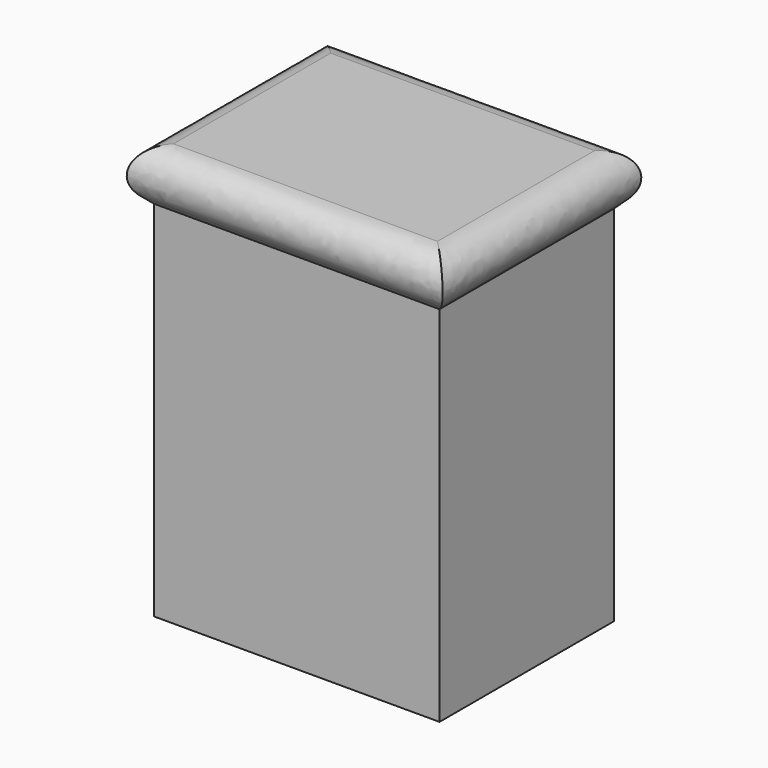
from build123d import *

# Parameters (mm, degrees)
F0_W      = 5.5
F0_H      = 4.2
F1_DEPTH  = 7
F2_W      = 0.8
F2_H      = 0.95
F3_DEPTH  = 5
F1_FACE_W = 5.5
F1_FACE_H = 4.2
F4_DEPTH  = 1
F4_TAPER  = -45
F6_R      = 0.5


# Not quite as in the source:
# - a feature of the source that left no trace in its solid (it failed there, or was rolled back) is left out


with BuildPart() as f1:
    # F0 (on Top) → F1 (new body)
    with BuildSketch(Plane.XY):
        Rectangle(F0_W, F0_H)
    extrude(amount=F1_DEPTH)

    # F2 (on Top) → F3 (cut)
    with BuildSketch(Plane.XY):
        with Locations((-1.2, 0)):
            Rectangle(F2_W, F2_H)
    extrude(amount=F3_DEPTH, mode=Mode.SUBTRACT)

    # F1_face (on face) → F4 (join)
    with BuildSketch(Plane.XY.offset(7)):
        Rectangle(F1_FACE_W, F1_FACE_H)
    extrude(amount=F4_DEPTH, taper=F4_TAPER)

    # F6
    f6_edges = [f1.edges().sort_by_distance(p)[0] for p in [
        (0, -3.1, 8),
        (3.75, 0, 8),
        (0, 3.1, 8),
        (-3.75, 0, 8),
    ]]
    fillet(f6_edges, radius=F6_R)


solid = f1.part
